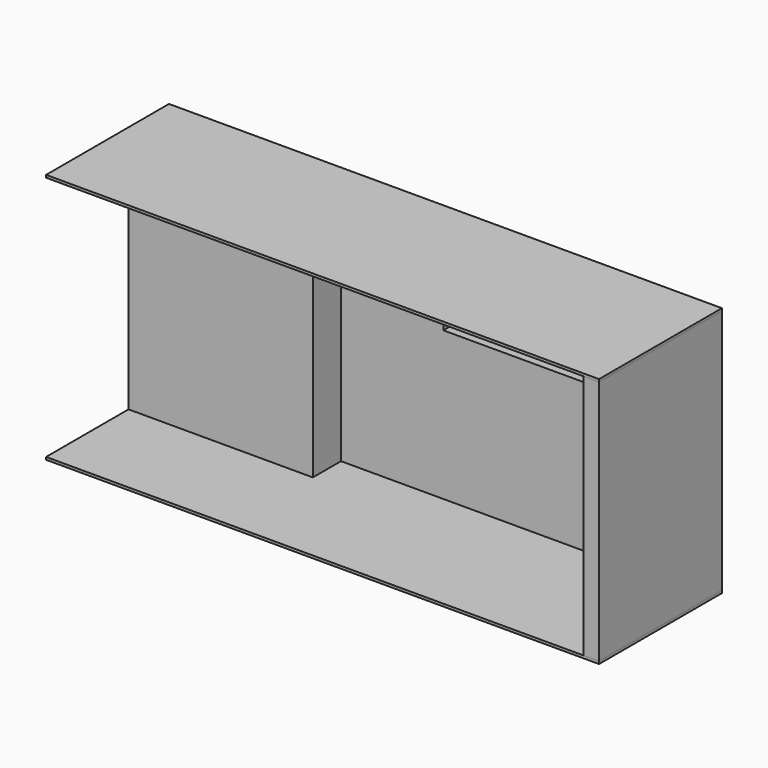
from build123d import *

# Parameters (mm, degrees)
F0_W      = 3505.2
F0_H      = 2438.4
F0_W_2    = 1466.85
F0_H_2    = 577.85
F1_DEPTH  = 152.4
F2_W      = 349.25
F2_H      = 2438.4
F1_FACE_W = 152.4
F1_FACE_H = 2438.4
F3_DEPTH  = 1828.8
F4_W      = 1371.6
F4_H      = 2438.4
F4_W_2    = 152.4
F5_DEPTH  = 152.4
F7_DEPTH  = 25.4
F8_W      = 5486.4
F8_H      = 1524
F9_DEPTH  = 25.4


with BuildPart() as f1:
    # F0 (on Front) → F1 (new body)
    with BuildSketch(Plane.XZ):
        with Locations((1752.6, 1219.2)):
            Rectangle(F0_W, F0_H)
        with Locations((1749.425, 1762.125)):
            Rectangle(F0_W_2, F0_H_2, mode=Mode.SUBTRACT)
    extrude(amount=-F1_DEPTH)

    # F2 (on Right) + F1_face (on face) → F3 (join)
    with BuildSketch(Plane.YZ):
        with Locations((-174.625, 1219.2)):
            Rectangle(F2_W, F2_H)
    with BuildSketch(Plane(origin=(0, 76.2, 1219.2), x_dir=(0, -1, 0), z_dir=(-1, 0, 0))):
        Rectangle(F1_FACE_W, F1_FACE_H)
    extrude(amount=-F3_DEPTH, dir=(1, 0, 0))

    # F4 (on face) → F5 (join)
    with BuildSketch(Plane.YZ.offset(3505.2)):
        with Locations((-685.8, 1219.2)):
            Rectangle(F4_W, F4_H)
        with Locations((76.2, 1219.2)):
            Rectangle(F4_W_2, F4_H)
    extrude(amount=F5_DEPTH)


with BuildPart() as f7:
    # F6 (on face) → F7 (new body)
    with BuildSketch(Plane.XY.offset(2438.4)):
        Polygon((-1828.8, -1371.6), (3505.2, -1371.6), (3505.2, 0), (0, 0), (0, -349.25), (-1828.8, -349.25), align=None)
        Polygon((3657.6, -1371.6), (3657.6, 152.4), (-1828.8, 152.4), (-1828.8, -349.25), (0, -349.25), (0, 0), (3505.2, 0), (3505.2, -1371.6), align=None)
    extrude(amount=F7_DEPTH)


with BuildPart() as f9:
    # F8 (on Top) → F9 (new body)
    with BuildSketch(Plane.XY):
        with Locations((914.4, -609.6)):
            Rectangle(F8_W, F8_H)
    extrude(amount=-F9_DEPTH)


solid = Compound([f1.part, f7.part, f9.part])
